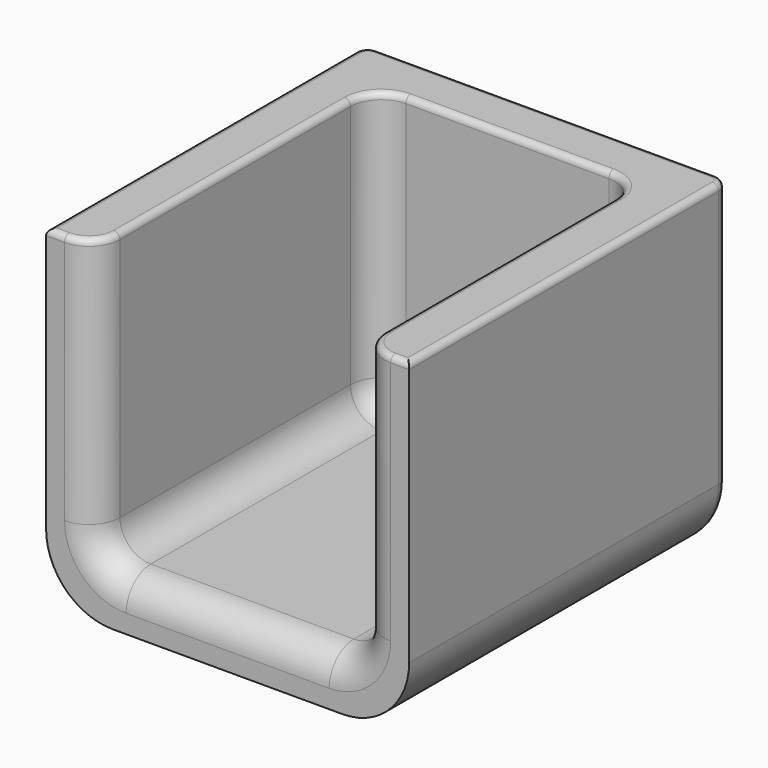
from build123d import *

# Parameters (mm, degrees)
F0_W     = 58.9698813856
F0_H     = 53.7666678429
F1_DEPTH = 32.4
F2_T     = -8
F3_R     = 5
F4_R     = 10.8639610307
F5_R     = 2
F6_R     = 1
F7_R     = 2.5
F8_DEPTH = 1


with BuildPart() as f1:
    # F0 (on Front) → F1 (new body, symmetric)
    with BuildSketch(Plane.XZ):
        Rectangle(F0_W, F0_H)
    extrude(amount=F1_DEPTH, both=True)

    # F2
    f2_openings = [f1.faces().sort_by_distance(p)[0] for p in [
        (0, 0, 26.883334),
        (0, -32.4, 0),
    ]]
    offset(amount=F2_T, openings=f2_openings)

    # F3
    f3_edges = [f1.edges().sort_by_distance(p)[0] for p in [
        (0, 24.4, -18.883334),
        (0, -32.4, -18.883334),
        (-21.484941, -4, -18.883334),
        (21.484941, -4, -18.883334),
        (-21.484941, 24.4, 4),
        (21.484941, 24.4, 4),
        (21.484941, -32.4, 4),
        (-21.484941, -32.4, 4),
    ]]
    fillet(f3_edges, radius=F3_R)

    # F4
    f4_edges = [f1.edges().sort_by_distance(p)[0] for p in [
        (29.484941, 0, -26.883334),
        (-29.484941, 0, -26.883334),
    ]]
    fillet(f4_edges, radius=F4_R)

    # F5
    f5_edges = [f1.edges().sort_by_distance(p)[0] for p in [
        (0, 32.4, -26.883334),
        (29.484941, 32.4, 5.431981),
        (26.30296, 32.4, -23.701353),
        (-26.30296, 32.4, -23.701353),
        (-29.484941, 32.4, 5.431981),
    ]]
    fillet(f5_edges, radius=F5_R)

    # F6
    f6_edges = [f1.edges().sort_by_distance(p)[0] for p in [
        (0, 24.4, 26.883334),
        (29.484941, -1, 26.883334),
        (28.899154, 31.814214, 26.883334),
        (27.984941, -32.4, 26.883334),
        (-27.984941, -32.4, 26.883334),
        (0, 32.4, 26.883334),
        (22.949407, -30.935534, 26.883334),
        (-28.899154, 31.814214, 26.883334),
        (21.484941, -4, 26.883334),
        (-29.484941, -1, 26.883334),
        (20.020475, 22.935534, 26.883334),
        (-22.949407, -30.935534, 26.883334),
        (-20.020475, 22.935534, 26.883334),
        (-21.484941, -4, 26.883334),
    ]]
    fillet(f6_edges, radius=F6_R)

    # F7 (on face) → F8 (cut)
    with BuildSketch(Plane(origin=(0, 0, -26.8833339214), x_dir=(1, 0, 0), z_dir=(0, 0, -1))):
        Circle(F7_R)
    extrude(amount=-F8_DEPTH, mode=Mode.SUBTRACT)


solid = f1.part
